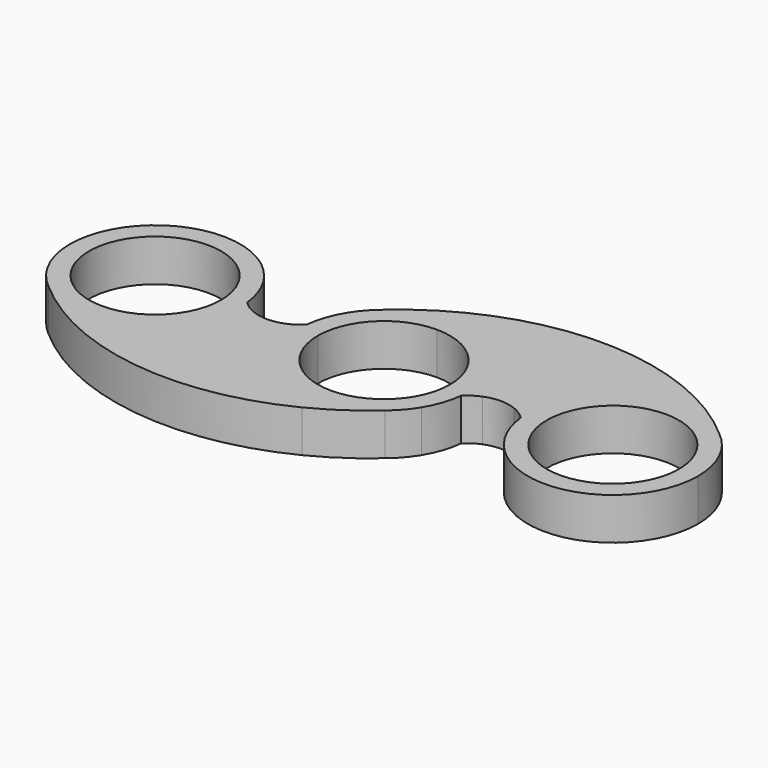
from build123d import *

# Parameters (mm, degrees)
F0_R     = 11
F1_DEPTH = 7


# Not quite as in the source:
# - a feature names something its author has since deleted; it is built from what else it names


with BuildPart() as f1:
    # F0 (on Top) → F1 (new body)
    with BuildSketch(Plane.XY):
        with BuildLine():
            Line((14.175, 0), (11, 0))
            ThreePointArc((11, 0), (7.7781745931, -7.7781745931), (0, -11))
            Line((0, -11), (0, -14.175))
            ThreePointArc((0, -14.175), (4.7450574285, -13.3572098509), (8.9426071008, -10.9982))
            ThreePointArc((8.9426071008, -10.9982), (10.6919977036, -9.3065466262), (12.1262614453, -7.3406))
            ThreePointArc((12.1262614453, -7.3406), (12.4422930723, -4.2253938225), (14.0886784217, -1.561974817))
            ThreePointArc((14.0886784217, -1.561974817), (14.1534031531, -0.7821791265), (14.175, 0))
        make_face()
        with BuildLine():
            ThreePointArc((0, 11), (7.7781745931, 7.7781745931), (11, 0))
            Line((11, 0), (14.175, 0))
            ThreePointArc((14.175, 0), (10.0232386233, 10.0232386233), (0, 14.175))
            Line((0, 14.175), (0, 11))
        make_face()
        with BuildLine():
            ThreePointArc((-11, 0), (-7.7781745931, 7.7781745931), (0, 11))
            Line((0, 11), (0, 14.175))
            ThreePointArc((0, 14.175), (-4.7437129445, 13.3576873934), (-8.9403928885, 11))
            ThreePointArc((-8.9403928885, 11), (-10.6938487189, 9.304419626), (-12.1306573285, 7.3333333333))
            ThreePointArc((-12.1306573285, 7.3333333333), (-12.4461611466, 4.2234349909), (-14.0884789594, 1.5637728768))
            ThreePointArc((-14.0884789594, 1.5637728768), (-14.1533532113, 0.7830822914), (-14.175, 0))
            Line((-14.175, 0), (-11, 0))
        make_face()
        with BuildLine():
            Line((0, -14.175), (0, -11))
            ThreePointArc((0, -11), (-7.7781745931, -7.7781745931), (-11, 0))
            Line((-11, 0), (-14.175, 0))
            ThreePointArc((-14.175, 0), (-10.0232386233, -10.0232386233), (0, -14.175))
        make_face()
        with BuildLine():
            ThreePointArc((0, 14.175), (10.0232386233, 10.0232386233), (14.175, 0))
            Line((14.175, 0), (16.4338, 0))
            ThreePointArc((16.4338, 0), (19.05, 0.5089718042), (21.6662, 0))
            Line((21.6662, 0), (23.925, 0))
            ThreePointArc((23.925, 0), (32.0102886216, 12.8002359481), (47.0426071008, 10.9982))
            ThreePointArc((47.0426071008, 10.9982), (24.4514597735, 21.2483327836), (0, 17.0589086472))
            Line((0, 17.0589086472), (0, 14.175))
        make_face()
        with BuildLine():
            Line((16.4338, 0), (14.175, 0))
            ThreePointArc((14.175, 0), (14.1534031531, -0.7821791265), (14.0886784217, -1.561974817))
            ThreePointArc((14.0886784217, -1.561974817), (15.1815830564, -0.6613930561), (16.4338, 0))
        make_face()
        with BuildLine():
            ThreePointArc((-8.9403928885, 11), (-4.7437129445, 13.3576873934), (0, 14.175))
            Line((0, 14.175), (0, 17.0589086472))
            ThreePointArc((0, 17.0589086472), (-4.6644934549, 14.3161547368), (-8.9403928885, 11))
        make_face()
        with BuildLine():
            Line((0, -17.0538866478), (0, -14.175))
            ThreePointArc((0, -14.175), (-10.0232386233, -10.0232386233), (-14.175, 0))
            Line((-14.175, 0), (-16.4338, 0))
            ThreePointArc((-16.4338, 0), (-19.05, -0.5093373751), (-21.6662, 0))
            Line((-21.6662, 0), (-23.925, 0))
            ThreePointArc((-23.925, 0), (-32.0102886216, -12.8002359481), (-47.0426071008, -10.9982))
            ThreePointArc((-47.0426071008, -10.9982), (-24.4500361697, -21.2407501362), (0, -17.0538866478))
        make_face()
        with BuildLine():
            ThreePointArc((8.9426071008, -10.9982), (4.7450574285, -13.3572098509), (0, -14.175))
            Line((0, -14.175), (0, -17.0538866478))
            ThreePointArc((0, -17.0538866478), (4.6653864802, -14.3126511831), (8.9426071008, -10.9982))
        make_face()
        with BuildLine():
            ThreePointArc((12.1262614453, -7.3406), (13.4221419792, -4.55814981), (14.0886784217, -1.561974817))
            ThreePointArc((14.0886784217, -1.561974817), (12.4422930723, -4.2253938225), (12.1262614453, -7.3406))
        make_face()
        with BuildLine():
            Line((-16.4338, 0), (-14.175, 0))
            ThreePointArc((-14.175, 0), (-14.1533532113, 0.7830822914), (-14.0884789594, 1.5637728768))
            ThreePointArc((-14.0884789594, 1.5637728768), (-15.1813037797, 0.6621501584), (-16.4338, 0))
        make_face()
        with BuildLine():
            Line((23.925, 0), (21.6662, 0))
            ThreePointArc((21.6662, 0), (22.9184169436, -0.6613930561), (24.0113215783, -1.561974817))
            ThreePointArc((24.0113215783, -1.561974817), (23.9465968469, -0.7821791265), (23.925, 0))
        make_face()
        with BuildLine():
            ThreePointArc((-12.1306573285, 7.3333333333), (-13.4232162274, 4.5549853033), (-14.0884789594, 1.5637728768))
            ThreePointArc((-14.0884789594, 1.5637728768), (-12.4461611466, 4.2234349909), (-12.1306573285, 7.3333333333))
        make_face()
        with BuildLine():
            ThreePointArc((52.275, 0), (50.9002359481, 6.0897113784), (47.0426071008, 10.9982))
            ThreePointArc((47.0426071008, 10.9982), (32.0102886216, 12.8002359481), (23.925, 0))
            ThreePointArc((23.925, 0), (23.9465968469, -0.7821791265), (24.0113215783, -1.561974817))
            ThreePointArc((24.0113215783, -1.561974817), (25.6577069277, -4.2253938225), (25.9737385547, -7.3406))
            ThreePointArc((25.9737385547, -7.3406), (41.9105687904, -13.6532117281), (52.275, 0))
        make_face()
        with BuildLine():
            ThreePointArc((49.1, 0), (38.1, -11), (27.1, 0))
            ThreePointArc((27.1, 0), (38.1, 11), (49.1, 0))
        make_face(mode=Mode.SUBTRACT)
        with BuildLine():
            ThreePointArc((-25.9693426715, 7.3333333333), (-47.4033431975, 10.6947851941), (-47.0426071008, -10.9982))
            ThreePointArc((-47.0426071008, -10.9982), (-32.0102886216, -12.8002359481), (-23.925, 0))
            ThreePointArc((-23.925, 0), (-23.9466467887, 0.7830822914), (-24.0115210406, 1.5637728768))
            ThreePointArc((-24.0115210406, 1.5637728768), (-25.6538388534, 4.2234349909), (-25.9693426715, 7.3333333333))
        make_face()
        with Locations((-38.1, 0)):
            Circle(F0_R, mode=Mode.SUBTRACT)
        with BuildLine():
            ThreePointArc((25.9737385547, -7.3406), (25.6577069277, -4.2253938225), (24.0113215783, -1.561974817))
            ThreePointArc((24.0113215783, -1.561974817), (24.6778580208, -4.55814981), (25.9737385547, -7.3406))
        make_face()
        with BuildLine():
            Line((-23.925, 0), (-21.6662, 0))
            ThreePointArc((-21.6662, 0), (-22.9186962203, 0.6621501584), (-24.0115210406, 1.5637728768))
            ThreePointArc((-24.0115210406, 1.5637728768), (-23.9466467887, 0.7830822914), (-23.925, 0))
        make_face()
        with BuildLine():
            ThreePointArc((-24.0115210406, 1.5637728768), (-24.6767837726, 4.5549853033), (-25.9693426715, 7.3333333333))
            ThreePointArc((-25.9693426715, 7.3333333333), (-25.6538388534, 4.2234349909), (-24.0115210406, 1.5637728768))
        make_face()
    extrude(amount=F1_DEPTH)


solid = f1.part
